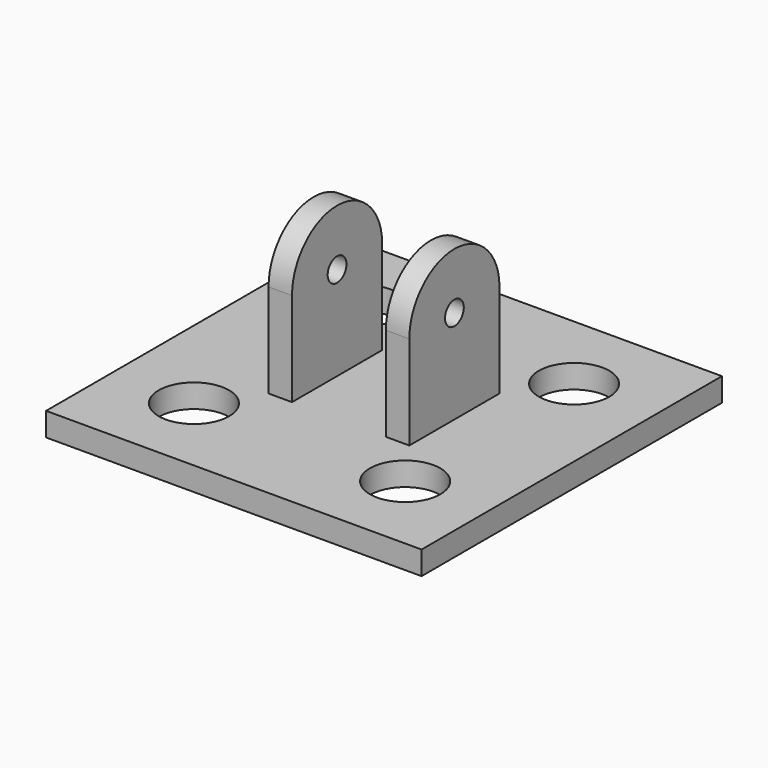
from build123d import *

# Parameters (mm, degrees)
F0_W     = 101.6
F0_H     = 101.6
F0_R     = 9.525
F1_DEPTH = 6.35
F2_W     = 6.35
F2_H     = 30.48
F3_DEPTH = 25.4
F4_W     = 6.35
F4_H     = 15.24
F7_R     = 3.175
F8_DEPTH = 44.45


with BuildPart() as f1:
    # F0 (on Top) → F1 (new body)
    with BuildSketch(Plane.XY):
        Rectangle(F0_W, F0_H)
        with Locations((-28.575, -28.575)):
            Circle(F0_R, mode=Mode.SUBTRACT)
        with Locations((28.575, -28.575)):
            Circle(F0_R, mode=Mode.SUBTRACT)
        with Locations((-28.575, 28.575)):
            Circle(F0_R, mode=Mode.SUBTRACT)
        with Locations((28.575, 28.575)):
            Circle(F0_R, mode=Mode.SUBTRACT)
    extrude(amount=F1_DEPTH)

    # F2 (on face) → F3 (join)
    with BuildSketch(Plane.XY.offset(6.35)):
        with Locations((15.875, 0)):
            Rectangle(F2_W, F2_H)
        with Locations((-15.875, 0)):
            Rectangle(F2_W, F2_H)
    extrude(amount=F3_DEPTH)

    # F4 (on face) → F5 (revolve)
    with BuildSketch(Plane.XY.offset(31.75)):
        with Locations((15.875, -7.62)):
            Rectangle(F4_W, F4_H)
    revolve(axis=Axis((15.875, 0, 31.75), (1, 0, 0)))

    # F6: F1 across plane


with BuildPart() as f1_1:
    add(f1.part)
    add(f1.part.mirror(Plane.YZ))

    # F7 (on face) → F8 (cut)
    with BuildSketch(Plane.YZ.offset(19.05)):
        with Locations((0, 31.75)):
            Circle(F7_R)
    extrude(amount=-F8_DEPTH, mode=Mode.SUBTRACT)


solid = f1_1.part
